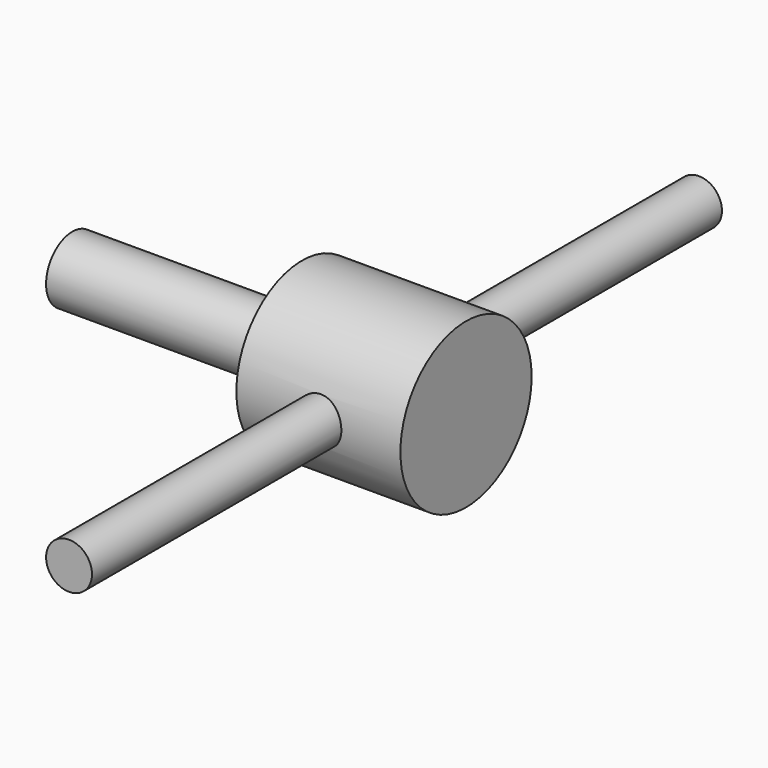
from build123d import *

# Parameters (mm, degrees)
F0_R     = 15.875
F1_DEPTH = 15.875
F2_R     = 6.35
F3_DEPTH = 44.45
F4_R     = 4.445
F5_DEPTH = 76.2


# Not quite as in the source:
# - the program builds the solid bodies; features that only make, move or delete a surface that nothing else refers to are left out


with BuildPart() as f1:
    # F0 (on Right) → F1 (new body, symmetric)
    with BuildSketch(Plane.YZ):
        Circle(F0_R)
    extrude(amount=F1_DEPTH, both=True)

    # F2 (on face) → F3 (join)
    with BuildSketch(Plane(origin=(-15.875, 0, 0), x_dir=(0, -1, 0), z_dir=(-1, 0, 0))):
        Circle(F2_R)
    extrude(amount=F3_DEPTH)

    # F4 (on Front) → F5 (join, symmetric)
    with BuildSketch(Plane.XZ):
        Circle(F4_R)
    extrude(amount=F5_DEPTH, both=True)


solid = f1.part
